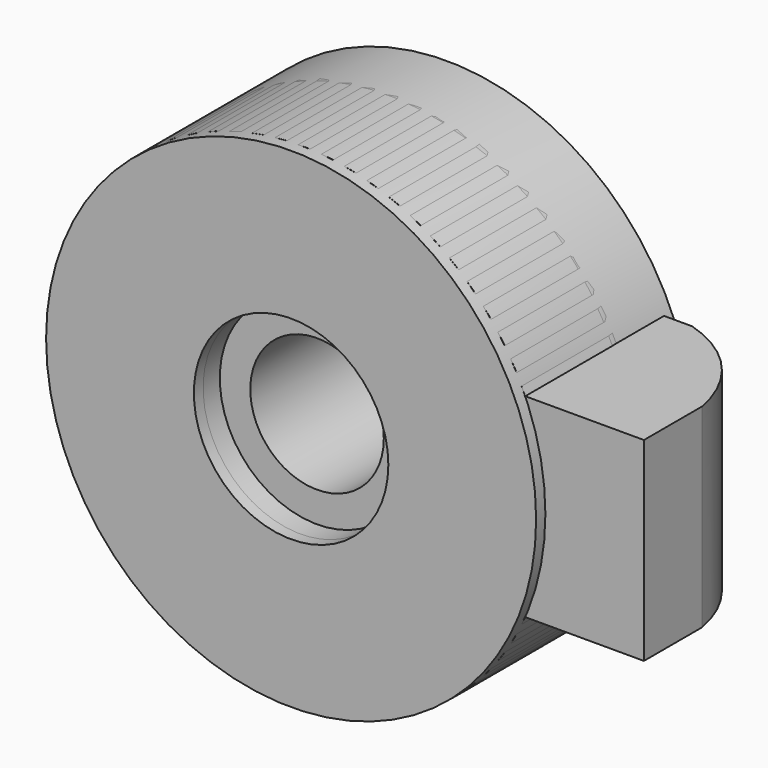
from build123d import *

# Parameters (mm, degrees)
F0_R     = 24.003
F0_R_2   = 9.525
F1_DEPTH = 9.525
F2_R     = 6.5405
F3_DEPTH = 6.35
F7_DEPTH = 9.525


with BuildPart() as f1:
    # F0 (on Front) → F1 (new body, symmetric)
    with BuildSketch(Plane.XZ):
        Circle(F0_R)
        Circle(F0_R_2, mode=Mode.SUBTRACT)
    extrude(amount=F1_DEPTH, both=True)


with BuildPart() as f3:
    # F2 (on Front) → F3 (new body, symmetric)
    with BuildSketch(Plane.XZ):
        with BuildLine():
            Line((4.7625, -24.765), (4.7625, -17.7885024313))
            ThreePointArc((4.7625, -17.7885024313), (0, 18.415), (-4.7625, -17.7885024313))
            Line((-4.7625, -17.7885024313), (-4.7625, -24.765))
            Line((-4.7625, -24.765), (4.7625, -24.765))
        make_face()
        Circle(F2_R, mode=Mode.SUBTRACT)
    extrude(amount=F3_DEPTH, both=True)


with BuildPart() as f5:
    # F4 (on Top) → F5 (revolve)
    with BuildSketch(Plane.XY):
        with BuildLine():
            Line((9.525, 2.2752935514), (9.525, -8.3927064486))
            Line((9.525, -8.3927064486), (24.003, -8.3927064486))
            Line((24.003, -8.3927064486), (24.003, 2.2752935514))
            ThreePointArc((24.003, 2.2752935514), (22.1431280605, 6.7654216119), (17.653, 8.6252935514))
            Line((17.653, 8.6252935514), (15.875, 8.6252935514))
            ThreePointArc((15.875, 8.6252935514), (11.3848719395, 6.7654216119), (9.525, 2.2752935514))
        make_face()
    revolve(axis=Axis((0, -0.6977617741, 0), (0, -1, 0)))

    # F6 (on Top) → F7 (join, symmetric)
    with BuildSketch(Plane.XY):
        with BuildLine():
            Line((24.765, 8.6252935514), (17.653, 8.6252935514))
            Line((17.653, 8.6252935514), (17.653, -8.3927064486))
            Line((17.653, -8.3927064486), (33.655, -8.3927064486))
            Line((33.655, -8.3927064486), (33.655, -1.2807064486))
            ThreePointArc((33.655, -1.2807064486), (30.6116739074, 4.9302060324), (24.765, 8.6252935514))
        make_face()
    extrude(amount=F7_DEPTH, both=True)


solid = Compound([f1.part, f3.part, f5.part])
